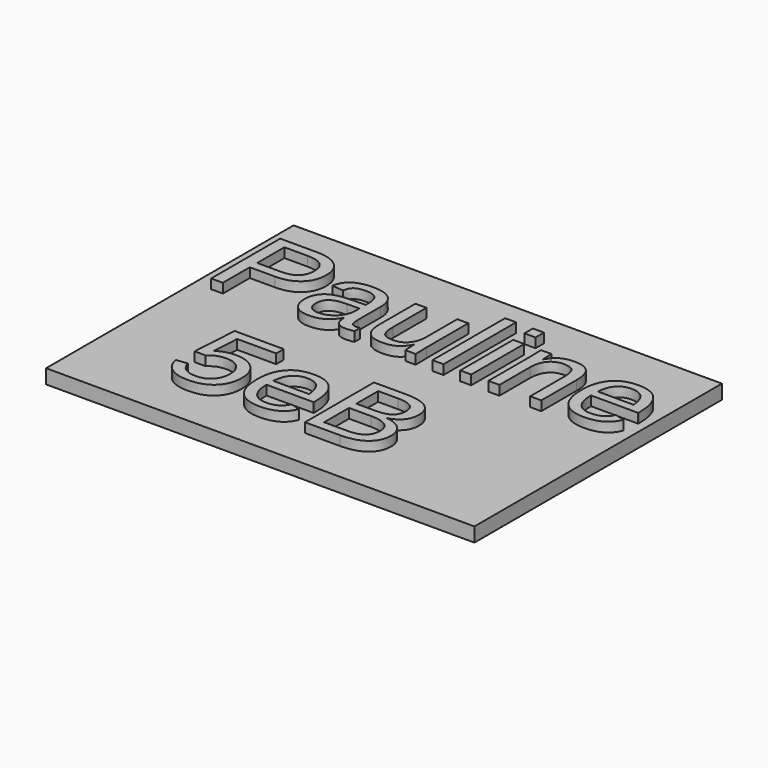
from build123d import *

# Parameters (mm, degrees)
F0_W         = 90
F0_H         = 65
F1_DEPTH     = 3
F2_TEXT_SIZE = 26.342050219
F3_DEPTH     = 2


# Not quite as in the source:
# - Text() gives the source's letters only with a copy of the font that has no kerning and outlines rounded to 1/6400 em; it was checked with that copy


with BuildPart() as f1:
    # F0 (on Top) → F1 (new body)
    with BuildSketch(Plane.XY):
        with Locations((45, -32.5)):
            Rectangle(F0_W, F0_H)
    extrude(amount=F1_DEPTH)

    # F2 (on face) → F3 (join)
    with BuildSketch(Plane.XY.offset(3)):
        with Locations((1.4701315375, -26.1731277493)):
            Text('Pauline', F2_TEXT_SIZE, font='Arimo', text_align=(TextAlign.LEFT, TextAlign.BOTTOM))
        with Locations((16.1064331904, -56.4664855012)):
            Text('5eB', F2_TEXT_SIZE, font='Arimo', text_align=(TextAlign.LEFT, TextAlign.BOTTOM))
    extrude(amount=F3_DEPTH)


solid = f1.part
